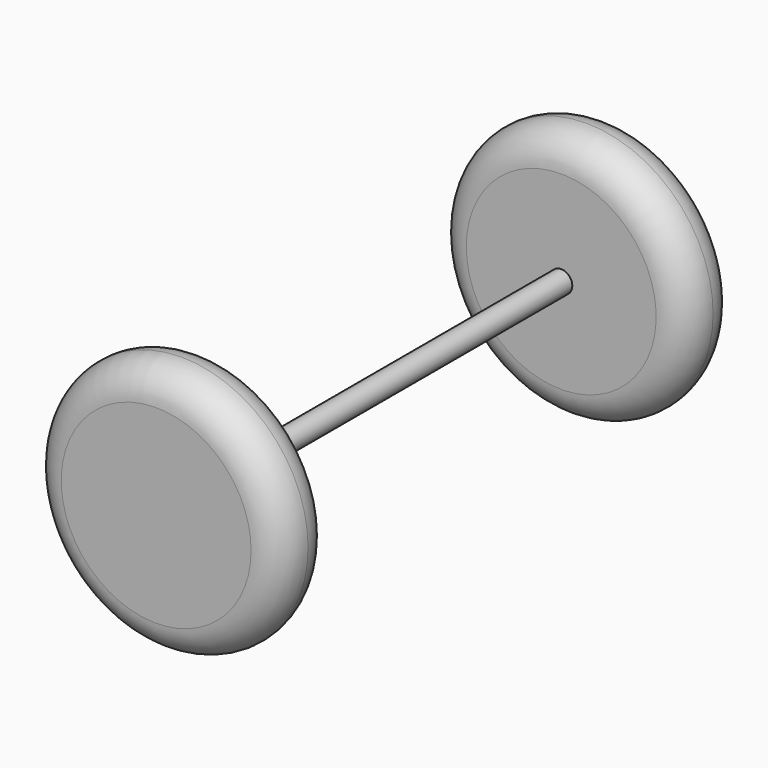
from build123d import *

# Parameters (mm, degrees)
F0_R     = 50.8
F1_DEPTH = 25.4
F2_R     = 12.7
F3_R     = 12.69999
F4_R     = 4.445
F5_DEPTH = 177.8
F6_R     = 50.8
F7_DEPTH = 25.4
F8_R     = 12.7
F9_R     = 12.69999


# Not quite as in the source:
# - a fillet or chamfer is up to 0.001 mm smaller than in the source, because OpenCascade refuses the exact size


with BuildPart() as f1:
    # F0 (on Front) → F1 (new body)
    with BuildSketch(Plane.XZ):
        Circle(F0_R)
    extrude(amount=F1_DEPTH)

    # F2
    f2_edges = [f1.edges().sort_by_distance(p)[0] for p in [
        (-50.8, -25.4, 0),
    ]]
    fillet(f2_edges, radius=F2_R)

    # F3 (radius 12.7 in the source; OpenCascade refuses exactly that, so slightly less here)
    f3_edges = [f1.edges().sort_by_distance(p)[0] for p in [
        (50.8, -6.35, 0),
        (-50.8, -12.7, 0),
        (-50.8, 0, 0),
    ]]
    fillet(f3_edges, radius=F3_R)

    # F4 (on face) → F5 (join)
    with BuildSketch(Plane(origin=(0, 0, 0), x_dir=(-1, 0, 0), z_dir=(0, 1, 0))):
        Circle(F4_R)
    extrude(amount=F5_DEPTH)

    # F6 (on face) → F7 (join)
    with BuildSketch(Plane(origin=(0, 177.8, 0), x_dir=(-1, 0, 0), z_dir=(0, 1, 0))):
        Circle(F6_R)
    extrude(amount=F7_DEPTH)

    # F8
    f8_edges = [f1.edges().sort_by_distance(p)[0] for p in [
        (50.8, 177.8, 0),
    ]]
    fillet(f8_edges, radius=F8_R)

    # F9 (radius 12.7 in the source; OpenCascade refuses exactly that, so slightly less here)
    f9_edges = [f1.edges().sort_by_distance(p)[0] for p in [
        (50.8, 203.2, 0),
    ]]
    fillet(f9_edges, radius=F9_R)


solid = f1.part
